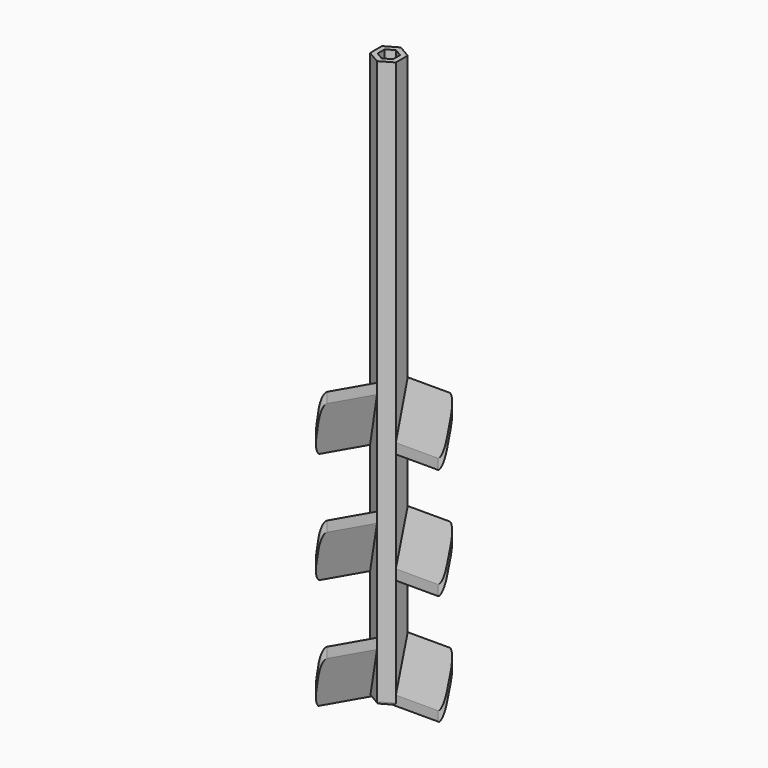
from build123d import *

# Parameters (mm, degrees)
F1_DEPTH     = 110
F3_DEPTH     = 9.14
F5_DEPTH     = 9.14
F7_DEPTH     = 9.14
F8_T1_DEPTH  = 8.75
F8_T3_DEPTH  = 8.75
F8_T5_DEPTH  = 8.75
F8_T7_DEPTH  = 8.75
F8_T9_DEPTH  = 8.75
F8_T11_DEPTH = 8.6204005009
F9_R         = 0.5


# Not quite as in the source:
# - a fillet or chamfer that OpenCascade refuses, or shapes differently, is made with other operations: its cross-section is extruded or revolved along the edge and cut away or added


with BuildPart() as f1:
    # F0 (on Top) → F1 (new body)
    with BuildSketch(Plane.XY):
        Polygon((2.5, 1.443375673), (0, 2.8867513459), (-2.5, 1.443375673), (-2.5, -1.443375673), (0, -2.8867513459), (2.5, -1.443375673), align=None)
        Polygon((-1.5, 0.8660254038), (0, 1.7320508076), (1.5, 0.8660254038), (1.5, -0.8660254038), (0, -1.7320508076), (-1.5, -0.8660254038), align=None, mode=Mode.SUBTRACT)
    extrude(amount=F1_DEPTH)

    # F2 (on face) → F3 (join)
    with BuildSketch(Plane(origin=(-1.25, -2.1650635095, 0), x_dir=(0.8660254038, -0.5, 0), z_dir=(-0.5, -0.8660254038, 0))):
        Polygon((-1.443375673, 43.018942656), (1.443375673, 53.018942656), (1.443375673, 55.018942656), (-1.443375673, 45.018942656), align=None)
        Polygon((1.443375673, 31.018942656), (1.443375673, 33.018942656), (-1.443375673, 23.4446715784), (-1.443375673, 21.4446715784), align=None)
        Polygon((1.443375673, 9.4446715784), (1.443375673, 11.4446715784), (-1.443375673, 1.8704005009), (-1.443375673, 0), (-1.4042999537, 0), align=None)
    extrude(amount=F3_DEPTH)

    # F4 (on face) → F5 (join)
    with BuildSketch(Plane(origin=(-1.25, 2.1650635095, 0), x_dir=(-0.8660254038, -0.5, 0), z_dir=(-0.5, 0.8660254038, 0))):
        Polygon((-1.443375673, 43.018942656), (1.443375673, 53.018942656), (1.443375673, 55.018942656), (-1.443375673, 45.018942656), align=None)
        Polygon((1.443375673, 31.018942656), (1.443375673, 33.018942656), (-1.443375673, 23.4446715784), (-1.443375673, 21.4446715784), align=None)
        Polygon((1.443375673, 9.4446715784), (1.443375673, 11.4446715784), (-1.443375673, 1.8704005009), (-1.443375673, 0), (-1.4042999537, 0), align=None)
    extrude(amount=F5_DEPTH)

    # F6 (on face) → F7 (join)
    with BuildSketch(Plane.YZ.offset(2.5)):
        Polygon((-1.443375673, 43.018942656), (1.443375673, 53.018942656), (1.443375673, 55.018942656), (-1.443375673, 45.018942656), align=None)
        Polygon((1.443375673, 31.018942656), (1.443375673, 33.018942656), (-1.443375673, 23.4446715784), (-1.443375673, 21.4446715784), align=None)
        Polygon((1.443375673, 9.4446715784), (1.443375673, 11.4446715784), (-1.443375673, 1.8704005009), (-1.443375673, 0), (-1.4042999537, 0), align=None)
    extrude(amount=F7_DEPTH)

    # F8: fillet of radius 1 on 18 edges, made by hand

    # F8_s2 → F8_t1 (cut)
    with BuildSketch(Plane.XY.offset(40.518942656)):
        with BuildLine():
            ThreePointArc((-6.57, -8.4928224598), (-6.6699004225, -9.2516415049), (-6.2039745962, -9.8588478636))
            Line((-6.2039745962, -9.8588478636), (-7.07, -9.3588478636))
            Line((-7.07, -9.3588478636), (-6.57, -8.4928224598))
        make_face()
        with BuildLine():
            ThreePointArc((11.64, -0.443375673), (11.3471067812, -1.1504824542), (10.64, -1.443375673))
            Line((10.64, -1.443375673), (11.64, -1.443375673))
            Line((11.64, -1.443375673), (11.64, -0.443375673))
        make_face()
        with BuildLine():
            ThreePointArc((-4.07, 9.9361981328), (-4.6772063587, 10.402123959), (-5.4360254038, 10.3022235365))
            Line((-5.4360254038, 10.3022235365), (-4.57, 10.8022235365))
            Line((-4.57, 10.8022235365), (-4.07, 9.9361981328))
        make_face()
    extrude(amount=F8_T1_DEPTH, mode=Mode.SUBTRACT)

    # F8_s4 → F8_t3 (cut)
    with BuildSketch(Plane.XY.offset(48.768942656)):
        with BuildLine():
            ThreePointArc((-4.07, -9.9361981328), (-4.6772063587, -10.402123959), (-5.4360254038, -10.3022235365))
            Line((-5.4360254038, -10.3022235365), (-4.57, -10.8022235365))
            Line((-4.57, -10.8022235365), (-4.07, -9.9361981328))
        make_face()
        with BuildLine():
            ThreePointArc((10.64, 1.443375673), (11.3471067812, 1.1504824542), (11.64, 0.443375673))
            Line((11.64, 0.443375673), (11.64, 1.443375673))
            Line((11.64, 1.443375673), (10.64, 1.443375673))
        make_face()
        with BuildLine():
            ThreePointArc((-6.2039745962, 9.8588478636), (-6.6699004225, 9.2516415049), (-6.57, 8.4928224598))
            Line((-6.57, 8.4928224598), (-7.07, 9.3588478636))
            Line((-7.07, 9.3588478636), (-6.2039745962, 9.8588478636))
        make_face()
    extrude(amount=F8_T3_DEPTH, mode=Mode.SUBTRACT)

    # F8_s6 → F8_t5 (cut)
    with BuildSketch(Plane.XY.offset(26.768942656)):
        with BuildLine():
            ThreePointArc((-4.07, -9.9361981328), (-4.6772063587, -10.402123959), (-5.4360254038, -10.3022235365))
            Line((-5.4360254038, -10.3022235365), (-4.57, -10.8022235365))
            Line((-4.57, -10.8022235365), (-4.07, -9.9361981328))
        make_face()
        with BuildLine():
            ThreePointArc((10.64, 1.443375673), (11.3471067812, 1.1504824542), (11.64, 0.443375673))
            Line((11.64, 0.443375673), (11.64, 1.443375673))
            Line((11.64, 1.443375673), (10.64, 1.443375673))
        make_face()
        with BuildLine():
            ThreePointArc((-6.2039745962, 9.8588478636), (-6.6699004225, 9.2516415049), (-6.57, 8.4928224598))
            Line((-6.57, 8.4928224598), (-7.07, 9.3588478636))
            Line((-7.07, 9.3588478636), (-6.2039745962, 9.8588478636))
        make_face()
    extrude(amount=F8_T5_DEPTH, mode=Mode.SUBTRACT)

    # F8_s8 → F8_t7 (cut)
    with BuildSketch(Plane.XY.offset(18.9446715784)):
        with BuildLine():
            ThreePointArc((-6.57, -8.4928224598), (-6.6699004225, -9.2516415049), (-6.2039745962, -9.8588478636))
            Line((-6.2039745962, -9.8588478636), (-7.07, -9.3588478636))
            Line((-7.07, -9.3588478636), (-6.57, -8.4928224598))
        make_face()
        with BuildLine():
            ThreePointArc((11.64, -0.443375673), (11.3471067812, -1.1504824542), (10.64, -1.443375673))
            Line((10.64, -1.443375673), (11.64, -1.443375673))
            Line((11.64, -1.443375673), (11.64, -0.443375673))
        make_face()
        with BuildLine():
            ThreePointArc((-4.07, 9.9361981328), (-4.6772063587, 10.402123959), (-5.4360254038, 10.3022235365))
            Line((-5.4360254038, 10.3022235365), (-4.57, 10.8022235365))
            Line((-4.57, 10.8022235365), (-4.07, 9.9361981328))
        make_face()
    extrude(amount=F8_T7_DEPTH, mode=Mode.SUBTRACT)

    # F8_s10 → F8_t9 (cut)
    with BuildSketch(Plane.XY.offset(5.1946715784)):
        with BuildLine():
            ThreePointArc((-5.4360254038, -10.3022235365), (-4.6772063587, -10.402123959), (-4.07, -9.9361981328))
            Line((-4.07, -9.9361981328), (-4.57, -10.8022235365))
            Line((-4.57, -10.8022235365), (-5.4360254038, -10.3022235365))
        make_face()
        with BuildLine():
            ThreePointArc((10.64, 1.443375673), (11.3471067812, 1.1504824542), (11.64, 0.443375673))
            Line((11.64, 0.443375673), (11.64, 1.443375673))
            Line((11.64, 1.443375673), (10.64, 1.443375673))
        make_face()
        with BuildLine():
            ThreePointArc((-6.2039745962, 9.8588478636), (-6.6699004225, 9.2516415049), (-6.57, 8.4928224598))
            Line((-6.57, 8.4928224598), (-7.07, 9.3588478636))
            Line((-7.07, 9.3588478636), (-6.2039745962, 9.8588478636))
        make_face()
    extrude(amount=F8_T9_DEPTH, mode=Mode.SUBTRACT)

    # F8_s12 → F8_t11 (cut)
    with BuildSketch(Plane.XY.offset(-2.5)):
        with BuildLine():
            ThreePointArc((-6.57, -8.4928224598), (-6.6699004225, -9.2516415049), (-6.2039745962, -9.8588478636))
            Line((-6.2039745962, -9.8588478636), (-7.07, -9.3588478636))
            Line((-7.07, -9.3588478636), (-6.57, -8.4928224598))
        make_face()
        with BuildLine():
            ThreePointArc((11.64, -0.443375673), (11.3471067812, -1.1504824542), (10.64, -1.443375673))
            Line((10.64, -1.443375673), (11.64, -1.443375673))
            Line((11.64, -1.443375673), (11.64, -0.443375673))
        make_face()
        with BuildLine():
            ThreePointArc((-4.07, 9.9361981328), (-4.6772063587, 10.402123959), (-5.4360254038, 10.3022235365))
            Line((-5.4360254038, 10.3022235365), (-4.57, 10.8022235365))
            Line((-4.57, 10.8022235365), (-4.07, 9.9361981328))
        make_face()
    extrude(amount=F8_T11_DEPTH, mode=Mode.SUBTRACT)

    # F9
    f9_edges = [f1.edges().sort_by_distance(p)[0] for p in [
        (1.25, -2.165064, 0),
        (-1.23308, -2.174832, 0),
        (-2.5, 0, 0),
        (-1.26692, 2.155295, 0),
        (1.25, 2.165064, 0),
        (2.5, 0.019538, 0),
    ]]
    fillet(f9_edges, radius=F9_R)


solid = f1.part
